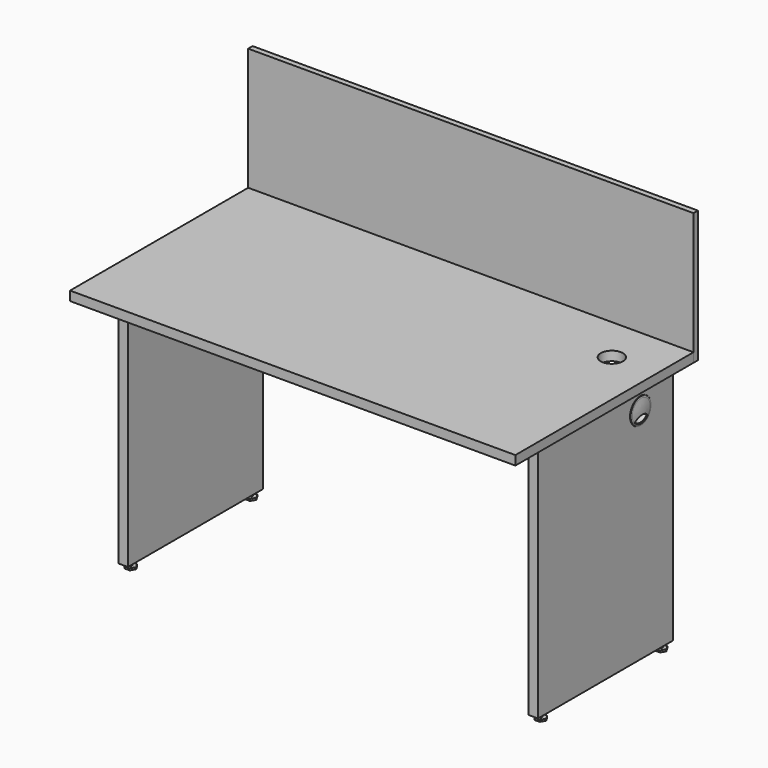
from build123d import *

# Parameters (mm, degrees)
F2_W      = 1200
F2_H      = 600
F2_R      = 30
F3_DEPTH  = 25
F5_W      = 455
F5_H      = 660
F5_R      = 30
F7_DEPTH  = 25
F13_DEPTH = 600.001
F14_R     = 2.5
F14_R_2   = 2
F15_DEPTH = 10
F16_R     = 4
F17_DEPTH = 10
F18_R     = 4
F19_DEPTH = 5
F20_DEPTH = 25
F22_W     = 1200
F22_H     = 355
F23_DEPTH = 15
F24_R     = 2
F25_DEPTH = 10


# Not quite as in the source:
# - a pattern or mirror of a feature is missing from the dataset's text; its kind, count and spacing are read off the source's solid


with BuildPart() as f3:
    # F2 (on Top) → F3 (new body)
    with BuildSketch(Plane.XY):
        Rectangle(F2_W, F2_H)
        with Locations((480, 175)):
            Circle(F2_R, mode=Mode.SUBTRACT)
    extrude(amount=-F3_DEPTH)

    # F14 (on face) → F15 (cut)
    with BuildSketch(Plane(origin=(0, 0, -25), x_dir=(1, 0, 0), z_dir=(0, 0, -1))):
        with Locations((533.5, 100)):
            Circle(F14_R)
        with Locations((533.5, -195)):
            Circle(F14_R)
        with Locations((500, -273)):
            Circle(F14_R_2)
    f15 = extrude(amount=-F15_DEPTH, mode=Mode.SUBTRACT)

    # F15_copies: F15 across plane
    add(f15.mirror(Plane(origin=(0, 0, 0), x_dir=(0, 0, -1), z_dir=(-1, 0, 0))), mode=Mode.SUBTRACT)


with BuildPart() as f7:
    # F5 (on offset) → F7 (new body)
    with BuildSketch(Plane.YZ.offset(565)):
        with Locations((47.5, -355)):
            Rectangle(F5_W, F5_H)
        with Locations((165, -95)):
            Circle(F5_R, mode=Mode.SUBTRACT)
    extrude(amount=-F7_DEPTH)

    # F16 (on face) → F17 (cut)
    with BuildSketch(Plane(origin=(0, 0, -685), x_dir=(1, 0, 0), z_dir=(0, 0, -1))):
        with Locations((552.5, 155)):
            Circle(F16_R)
        with Locations((552.5, -250)):
            Circle(F16_R)
    extrude(amount=-F17_DEPTH, mode=Mode.SUBTRACT)


with BuildPart() as f10:
    # F9 (on plane+point) → F10 (revolve)
    with BuildSketch(Plane.XZ.offset(-165)):
        Polygon((565, -65), (541, -65), (540, -66), (553, -66), (553, -67), (565, -67), (567, -65), (566, -60.5773502692), (565, -60), align=None)
    revolve(axis=Axis((547.4527119644, 165, -95), (1, 0, 0)))


with BuildPart() as f11:
    # F9 (on plane+point) → F11 (revolve)
    with BuildSketch(Plane.XZ.offset(-165)):
        with BuildLine():
            Line((565, -67), (553, -67))
            Line((553, -67), (552, -67))
            Line((552, -67), (552, -68.5))
            Line((552, -68.5), (565.632593262, -68.5))
            ThreePointArc((565.632593262, -68.5), (567.4069721213, -81.6972313534), (568, -95))
            Line((568, -95), (570, -95))
            ThreePointArc((570, -95), (569.2481343168, -79.9251865683), (567, -65))
            Line((567, -65), (565, -67))
        make_face()
    revolve(axis=Axis((547.4527119644, 165, -95), (1, 0, 0)))

    # F12 (on Right) → F13 (cut, through all)
    with BuildSketch(Plane.YZ):
        with BuildLine():
            ThreePointArc((142.5, -114.843134833), (165, -125), (187.5, -114.843134833))
            ThreePointArc((187.5, -114.843134833), (165, -103), (142.5, -114.843134833))
        make_face()
    extrude(amount=F13_DEPTH, mode=Mode.SUBTRACT)


with BuildPart() as f19:
    # F18 (on plane+point) → F19 (new body)
    with BuildSketch(Plane.XY.offset(-700)):
        Polygon((566.9337567297, -155), (559.7168783649, -142.5), (545.2831216351, -142.5), (538.0662432703, -155), (545.2831216351, -167.5), (559.7168783649, -167.5), align=None)
        with Locations((552.5, -155)):
            Circle(F18_R, mode=Mode.SUBTRACT)
        with Locations((552.5, -155)):
            Circle(F18_R)
    extrude(amount=F19_DEPTH)

    # F18 (on plane+point) → F20, piece 2 (join)
    with BuildSketch(Plane.XY.offset(-700)):
        with Locations((552.5, -155)):
            Circle(F18_R)
    extrude(amount=F20_DEPTH)


with BuildPart() as f19b:
    # F18 (on plane+point) → F19, piece 2 (new body)
    with BuildSketch(Plane.XY.offset(-700)):
        Polygon((566.9337567297, 250), (559.7168783649, 262.5), (545.2831216351, 262.5), (538.0662432703, 250), (545.2831216351, 237.5), (559.7168783649, 237.5), align=None)
        with Locations((552.5, 250)):
            Circle(F18_R, mode=Mode.SUBTRACT)
        with Locations((552.5, 250)):
            Circle(F18_R)
    extrude(amount=F19_DEPTH)

    # F18 (on plane+point) → F20 (join)
    with BuildSketch(Plane.XY.offset(-700)):
        with Locations((552.5, 250)):
            Circle(F18_R)
    extrude(amount=F20_DEPTH)


with BuildPart() as f21_1:
    # F21: instance of F10
    add(f10.part.mirror(Plane.YZ))


with BuildPart() as f21_2:
    # F21: instance of F7
    add(f7.part.mirror(Plane.YZ))


with BuildPart() as f21_3:
    # F21: instance of F11
    add(f11.part.mirror(Plane.YZ))


with BuildPart() as f21_4:
    # F21: instance of F19b
    add(f19b.part.mirror(Plane.YZ))


with BuildPart() as f21_5:
    # F21: instance of F19
    add(f19.part.mirror(Plane.YZ))


with BuildPart() as f23:
    # F22 (on face) → F23 (new body)
    with BuildSketch(Plane(origin=(0, 300, 0), x_dir=(-1, 0, 0), z_dir=(0, 1, 0))):
        with Locations((0, 152.5)):
            Rectangle(F22_W, F22_H)
    extrude(amount=F23_DEPTH)

    # F24 (on face) → F25 (cut)
    with BuildSketch(Plane(origin=(0, 0, -25), x_dir=(1, 0, 0), z_dir=(0, 0, -1))):
        with Locations((-500, -307.5)):
            Circle(F24_R)
        with BuildLine():
            ThreePointArc((500, -305.5), (498.5857864376, -308.9142135624), (502, -307.5))
            ThreePointArc((502, -307.5), (501.4142135624, -306.0857864376), (500, -305.5))
        make_face()
    extrude(amount=-F25_DEPTH, mode=Mode.SUBTRACT)


solid = Compound([f3.part, f7.part, f10.part, f11.part, f19.part, f19b.part, f21_1.part, f21_2.part, f21_3.part, f21_4.part, f21_5.part, f23.part])
